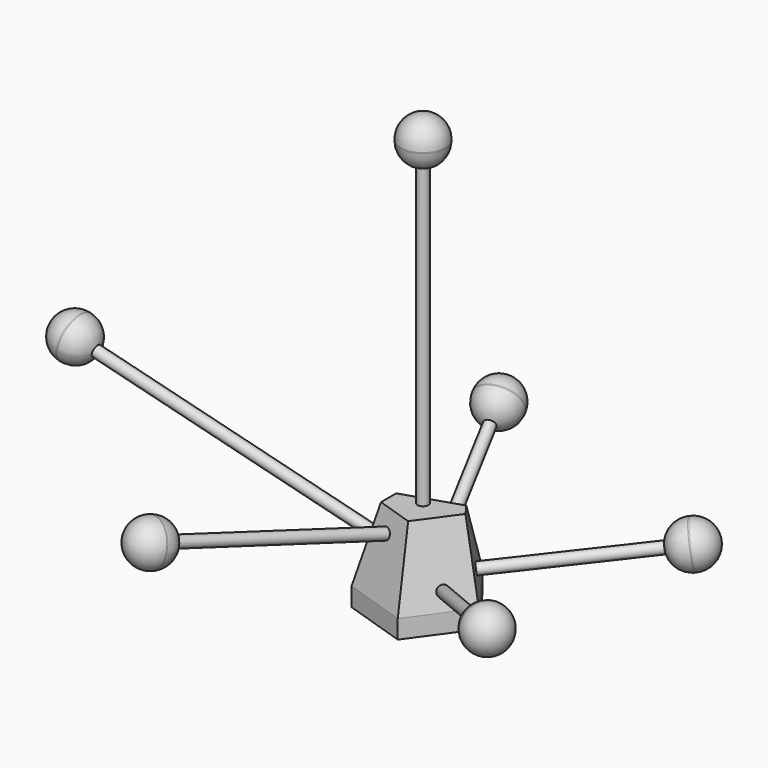
from build123d import *

# Parameters (mm, degrees)
F1_DEPTH    = 25
F2_SIZE2    = 5
F2_SIZE     = 20
F3_SIZE2    = 5
F3_SIZE     = 20
F4_SIZE2    = 3
F4_SIZE     = 20
F5_SIZE2    = 10
F5_SIZE     = 20
F6_T1_DEPTH = 105.7467241961
F7_R        = 1.5
F13_DEPTH   = 80
F8_R        = 1.5
F14_DEPTH   = 30
F9_R        = 1.5
F15_DEPTH   = 40
F10_R       = 1.5
F16_DEPTH   = 30
F11_R       = 1.5
F17_DEPTH   = 80
F12_R       = 1.5
F18_DEPTH   = 55
F19_R       = 6
F25_DEPTH   = 12
F20_R       = 6
F26_DEPTH   = 12
F21_R       = 6
F27_DEPTH   = 12
F22_R       = 6
F28_DEPTH   = 12
F23_R       = 6
F29_DEPTH   = 12
F24_R       = 6
F30_DEPTH   = 12
F31_R       = 6
F34_D       = 4
F34_DEPTH   = 4
F34_TIP     = 1.2017212381


# Not quite as in the source:
# - a fillet or chamfer that OpenCascade refuses, or shapes differently, is made with other operations: its cross-section is extruded or revolved along the edge and cut away or added


with BuildPart() as f1:
    # F0 (on Top) → F1 (new body)
    with BuildSketch(Plane.XY):
        Polygon((15, 0), (4.6352549156, 14.2658477444), (-12.1352549156, 8.8167787844), (-12.1352549156, -8.8167787844), (4.6352549156, -14.2658477444), align=None)
    extrude(amount=F1_DEPTH)

    # F2
    f2_edges = [f1.edges().sort_by_distance(p)[0] for p in [
        (-3.75, -11.541313, 25),
    ]]
    f2_side = f1.faces().sort_by_distance((-3.75, -11.541313, 12.5))[0]
    chamfer(f2_edges, length=F2_SIZE, length2=F2_SIZE2, reference=f2_side)

    # F3
    f3_edges = [f1.edges().sort_by_distance(p)[0] for p in [
        (11.362712, -5.006297, 25),
    ]]
    f3_side = f1.faces().sort_by_distance((10.379872, -6.359061, 11.710138))[0]
    chamfer(f3_edges, length=F3_SIZE, length2=F3_SIZE2, reference=f3_side)

    # F4
    f4_edges = [f1.edges().sort_by_distance(p)[0] for p in [
        (8.272542, 9.259551, 25),
    ]]
    f4_side = f1.faces().sort_by_distance((9.255383, 7.906786, 11.710138))[0]
    chamfer(f4_edges, length=F4_SIZE, length2=F4_SIZE2, reference=f4_side)

    # F5
    f5_edges = [f1.edges().sort_by_distance(p)[0] for p in [
        (-5.25, 11.053934, 25),
    ]]
    f5_side = f1.faces().sort_by_distance((-4.319172, 11.356378, 12.050432))[0]
    chamfer(f5_edges, length=F5_SIZE, length2=F5_SIZE2, reference=f5_side)

    # F6: chamfer of 20 x 5 on 1 edges, made by hand

    # F6_s2 → F6_t1 (cut)
    with BuildSketch(Plane.XZ.offset(-50.2447065374)):
        Polygon((-12.1352549156, 5), (-7.1352549156, 25), (-12.1352549156, 25), align=None)
    extrude(amount=F6_T1_DEPTH, mode=Mode.SUBTRACT)

    # F7 (on face) → F13 (join)
    with BuildSketch(Plane(origin=(-12.5978869794, 0, 3.1494717449), x_dir=(0, -1, 0), z_dir=(-0.9701425001, 0, 0.242535625))):
        with Locations((0, 10.203753598)):
            Circle(F7_R)
    extrude(amount=F13_DEPTH)

    # F8 (on face) → F14 (join)
    with BuildSketch(Plane(origin=(-3.6180339887, 11.1351636441, 5.8541019662), x_dir=(-0.9610446388, -0.2446443083, -0.1286171243), z_dir=(-0.2763932023, 0.8506508084, 0.4472135955))):
        with Locations((-3.206722904, 8.4386551753)):
            Circle(F8_R)
    extrude(amount=F14_DEPTH)

    # F9 (on face) → F15 (join)
    with BuildSketch(Plane(origin=(10.1950026441, 7.4071029941, 1.8902574448), x_dir=(-0.5715412914, 0.8137020337, -0.1059695832), z_dir=(0.8000663158, 0.5812822037, 0.1483404529))):
        with Locations((-2.0448169671, 8.4398761392)):
            Circle(F9_R)
    extrude(amount=F15_DEPTH)

    # F10 (on face) → F16 (join)
    with BuildSketch(Plane(origin=(10.1919046596, -7.4048521765, 3.1494717449), x_dir=(0.5448158193, 0.8214813003, 0.168357347), z_dir=(0.7848617696, -0.5702354542, 0.242535625))):
        with Locations((2.4632040877, 6.1464309692)):
            Circle(F10_R)
    extrude(amount=F16_DEPTH)

    # F11 (on face) → F17 (join)
    with BuildSketch(Plane.XY.offset(25)):
        Circle(F11_R)
    extrude(amount=F17_DEPTH)

    # F12 (on face) → F18 (join)
    with BuildSketch(Plane(origin=(-3.8929611699, -11.9813025033, 3.1494717449), x_dir=(0.9540050547, -0.2899406279, 0.0762154044), z_dir=(-0.2997905195, -0.9226603465, 0.242535625))):
        with Locations((0, 17.0320216566)):
            Circle(F12_R)
    extrude(amount=F18_DEPTH)

    # F19 (on face) → F25 (join)
    with BuildSketch(Plane(origin=(-20.3814397429, -62.7276215607, 16.4889311219), x_dir=(0.9540050547, -0.2899406279, 0.0762154044), z_dir=(-0.2997905195, -0.9226603465, 0.242535625))):
        with Locations((0, 17.0320216566)):
            Circle(F19_R)
    extrude(amount=F25_DEPTH)

    # F20 (on face) → F26 (join)
    with BuildSketch(Plane(origin=(33.737757747, -24.5119158028, 10.4255404959), x_dir=(0.5448158193, 0.8214813003, 0.168357347), z_dir=(0.7848617696, -0.5702354542, 0.242535625))):
        with Locations((2.4632040877, 6.1464309692)):
            Circle(F20_R)
    extrude(amount=F26_DEPTH)

    # F21 (on face) → F27 (join)
    with BuildSketch(Plane(origin=(42.1976552771, 30.6583911409, 7.823875562), x_dir=(-0.5715412914, 0.8137020337, -0.1059695832), z_dir=(0.8000663158, 0.5812822037, 0.1483404529))):
        with Locations((-2.0448169671, 8.4398761392)):
            Circle(F21_R)
    extrude(amount=F27_DEPTH)

    # F22 (on face) → F28 (join)
    with BuildSketch(Plane(origin=(-11.9098300563, 36.6546878947, 19.2705098312), x_dir=(-0.9610446388, -0.2446443083, -0.1286171243), z_dir=(-0.2763932023, 0.8506508084, 0.4472135955))):
        with Locations((-3.206722904, 8.4386551753)):
            Circle(F22_R)
    extrude(amount=F28_DEPTH)

    # F23 (on face) → F29 (join)
    with BuildSketch(Plane(origin=(-90.209286991, 0, 22.5523217478), x_dir=(0, -1, 0), z_dir=(-0.9701425001, 0, 0.242535625))):
        with Locations((0, 10.203753598)):
            Circle(F23_R)
    extrude(amount=F29_DEPTH)

    # F24 (on face) → F30 (join)
    with BuildSketch(Plane.XY.offset(105)):
        Circle(F24_R)
    extrude(amount=F30_DEPTH)

    # F31
    f31_edges = [f1.edges().sort_by_distance(p)[0] for p in [
        (-99.376223, 6, 35.361844),
        (-6.378477, 45.188017, 33.290534),
        (-6, 0, 117),
        (54.85778, 31.087694, 18.754911),
        (-29.702956, -67.72987, 35.414485),
        (39.414513, -34.260153, 18.612961),
    ]]
    fillet(f31_edges, radius=F31_R)

    # F32: fillet of radius 5.9 on 6 edges, made by hand

    # F32_s1 → F32_t2 (revolve, cut)
    with BuildSketch(Plane(origin=(0, -3.9268533113, 7.4693188604), x_dir=(1, 0, 0), z_dir=(0, 0.4653411272, -0.8851314226))):
        with BuildLine():
            ThreePointArc((-10.2695931595, -41.8833034178), (-13.9610472636, -42.9942942584), (-16.1784394484, -46.1477536208))
            Line((-16.1784394484, -46.1477536208), (-14.594294034, -40.6395340077))
            Line((-14.594294034, -40.6395340077), (-10.2695931595, -41.8833034178))
        make_face()
    revolve(axis=Axis((-8.8280262013, 33.5123410902, 27.15226817), (-0.2763932023, 0.8506508084, 0.4472135955)), mode=Mode.SUBTRACT)

    # F32_s3 → F32_t4 (revolve, cut)
    with BuildSketch(Plane(origin=(-1.5386160993, 0, 8.2984438146), x_dir=(0, 1, 0), z_dir=(0.1823031611, 0, -0.9832423696))):
        with BuildLine():
            ThreePointArc((30.2150724668, 43.2335322221), (34.0656604389, 43.0488532565), (37.208345891, 45.2814889635))
            Line((37.208345891, 45.2814889635), (33.8767316186, 40.6177623056))
            Line((33.8767316186, 40.6177623056), (30.2150724668, 43.2335322221))
        make_face()
    revolve(axis=Axis((41.8277365078, 28.9945194162, 16.3390077783), (0.8000663158, 0.5812822037, 0.1483404529)), mode=Mode.SUBTRACT)

    # F32_s5 → F32_t6 (revolve, cut)
    with BuildSketch(Plane.XZ):
        with BuildLine():
            ThreePointArc((6, 110.7314919524), (4.7405818601, 107.0880046119), (1.5, 105))
            Line((1.5, 105), (6, 105))
            Line((6, 105), (6, 110.7314919524))
        make_face()
    revolve(axis=Axis((0, 0, 105), (0, 0, 1)), mode=Mode.SUBTRACT)

    # F32_s7 → F32_t8 (revolve, cut)
    with BuildSketch(Plane(origin=(-1.8146833973, 0, 5.8724388313), x_dir=(0, 1, 0), z_dir=(0.2952418088, 0, -0.9554225632))):
        with BuildLine():
            ThreePointArc((-21.2562177554, 37.5718299013), (-19.7847946135, 41.1349813138), (-20.8278518207, 44.8462029069))
            Line((-20.8278518207, 44.8462029069), (-17.559551904, 40.1378894452))
            Line((-17.559551904, 40.1378894452), (-21.2562177554, 37.5718299013))
        make_face()
    revolve(axis=Axis((33.2650669029, -22.4884397059, 16.7126778325), (0.7848617696, -0.5702354542, 0.242535625)), mode=Mode.SUBTRACT)

    # F32_s9 → F32_t10 (revolve, cut)
    with BuildSketch(Plane(origin=(0, 4.3300315839, 16.4724190146), x_dir=(1, 0, 0), z_dir=(0, -0.2542288679, -0.9671440858))):
        with BuildLine():
            ThreePointArc((-18.9504321609, 65.3082962809), (-16.4848646735, 68.2717589543), (-16.3756563646, 72.1252259123))
            Line((-16.3756563646, 72.1252259123), (-14.6574094147, 66.6573536187))
            Line((-14.6574094147, 66.6573536187), (-18.9504321609, 65.3082962809))
        make_face()
    revolve(axis=Axis((-20.3814397429, -58.3975899768, 32.9613501365), (-0.2997905195, -0.9226603465, 0.242535625)), mode=Mode.SUBTRACT)

    # F32_s11 → F32_t12 (revolve, cut)
    with BuildSketch(Plane(origin=(2.4747737566, 0, 9.8990950265), x_dir=(0, 1, 0), z_dir=(-0.242535625, 0, -0.9701425001))):
        with BuildLine():
            ThreePointArc((-1.5, -92.9856046689), (-4.7405818601, -95.0736092808), (-6, -98.7170966213))
            Line((-6, -98.7170966213), (-6, -92.9856046689))
            Line((-6, -92.9856046689), (-1.5, -92.9856046689))
        make_face()
    revolve(axis=Axis((-87.7345132344, 0, 32.4514167742), (-0.9701425001, 0, 0.242535625)), mode=Mode.SUBTRACT)

    # F34
    with Locations(Plane(origin=(0, 0, 0), x_dir=(1, 0, 0), z_dir=(0, 0, -1))):
        with Locations((0, 0)):
            Hole(F34_D / 2, depth=F34_DEPTH)
            with Locations((0, 0, -(F34_DEPTH + F34_TIP / 2))):  # 118° drill point
                Cone(0, F34_D / 2, F34_TIP, mode=Mode.SUBTRACT)


solid = f1.part
